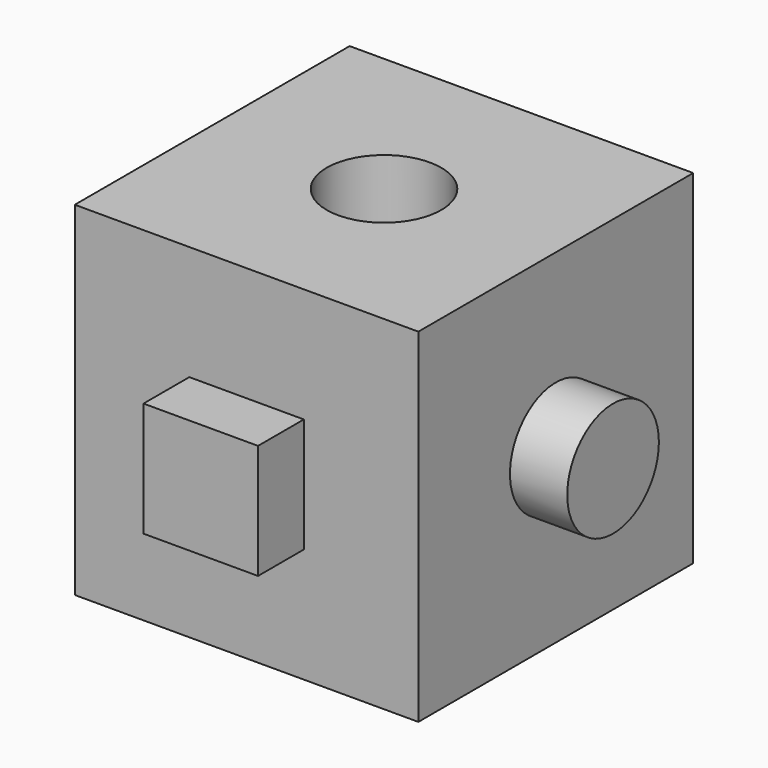
from build123d import *

# Parameters (mm, degrees)
F0_W     = 76.2
F0_H     = 76.2
F1_DEPTH = 76.2
F2_W     = 25.4
F2_H     = 25.4
F3_DEPTH = 12.7
F4_R     = 12.7
F5_DEPTH = 12.7
F7_D     = 25.4


# Not quite as in the source:
# - a length typed as a fraction of an inch, garbled in the dataset ("3 / 203.2 mm" for 3/8 in), is restored


with BuildPart() as f1:
    # F0 (on Front) → F1 (new body)
    with BuildSketch(Plane.XZ):
        with Locations((-8.3192586899, 10.8599686285)):
            Rectangle(F0_W, F0_H)
    extrude(amount=F1_DEPTH)

    # F2 (on face) → F3 (join)
    with BuildSketch(Plane.XZ.offset(76.2)):
        with Locations((-8.3192586899, 10.8599686285)):
            Rectangle(F2_W, F2_H)
    extrude(amount=F3_DEPTH)

    # F4 (on face) → F5 (join)
    with BuildSketch(Plane.YZ.offset(29.7807413101)):
        with Locations((-38.1, 10.8599686285)):
            Circle(F4_R)
    extrude(amount=F5_DEPTH)

    # F7 (through all)
    with Locations(Plane.XY.offset(48.9599686285)):
        with Locations((-8.3192586899, -38.1)):
            Hole(F7_D / 2)


solid = f1.part
